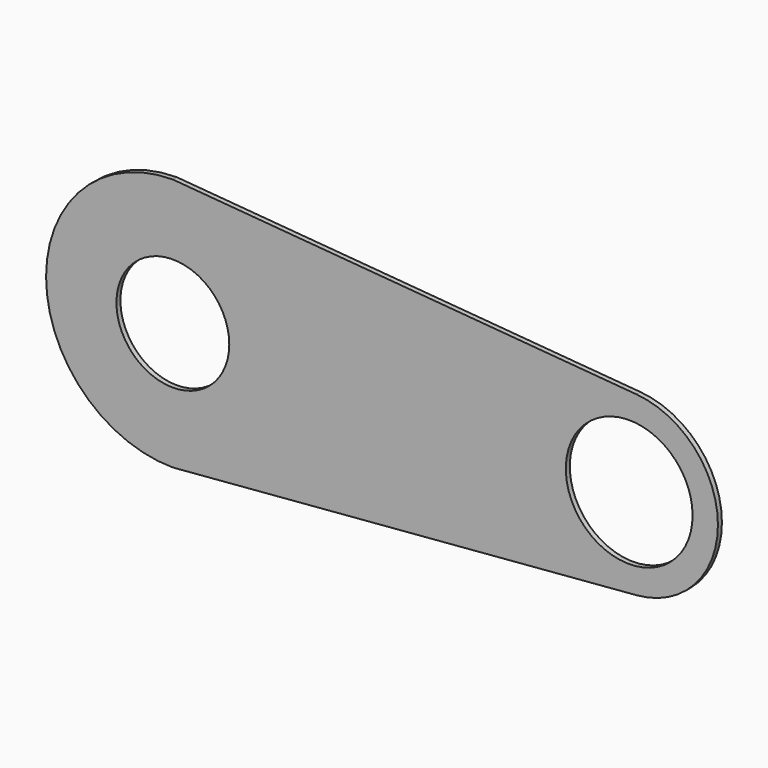
from build123d import *

# Parameters (mm, degrees)
F0_R     = 282.6342486107
F0_R_2   = 317.5
F1_DEPTH = 25


with BuildPart() as f1:
    # F0 (on Front) → F1 (new body)
    with BuildSketch(Plane.XZ):
        with BuildLine():
            Line((104.2782479982, 626.3793155863), (0, 635))
            ThreePointArc((0, 635), (-635, 0), (0, -635))
            Line((0, -635), (104.2782479982, -626.3793155863))
            ThreePointArc((104.2782479982, -626.3793155863), (484.4799724854, -410.492577595), (635, 0))
            ThreePointArc((635, 0), (484.4799724854, 410.492577595), (104.2782479982, 626.3793155863))
        make_face()
        Circle(F0_R, mode=Mode.SUBTRACT)
        with BuildLine():
            Line((2322.6218920545, 442.9888113963), (104.2782479982, 626.3793155863))
            ThreePointArc((104.2782479982, 626.3793155863), (484.4799724854, 410.492577595), (635, 0))
            ThreePointArc((635, 0), (484.4799724854, -410.492577595), (104.2782479982, -626.3793155863))
            Line((104.2782479982, -626.3793155863), (2322.6218920545, -442.9888113963))
            ThreePointArc((2322.6218920545, -442.9888113963), (1841.5, 0), (2322.6218920545, 442.9888113963))
        make_face()
        with BuildLine():
            ThreePointArc((2730.5, 0), (2613.0005206557, 301.0828947165), (2322.6218920545, 442.9888113963))
            ThreePointArc((2322.6218920545, 442.9888113963), (1841.5, 0), (2322.6218920545, -442.9888113963))
            ThreePointArc((2322.6218920545, -442.9888113963), (2613.0005206557, -301.0828947165), (2730.5, 0))
        make_face()
        with Locations((2286, 0)):
            Circle(F0_R_2, mode=Mode.SUBTRACT)
    extrude(amount=F1_DEPTH)


solid = f1.part
